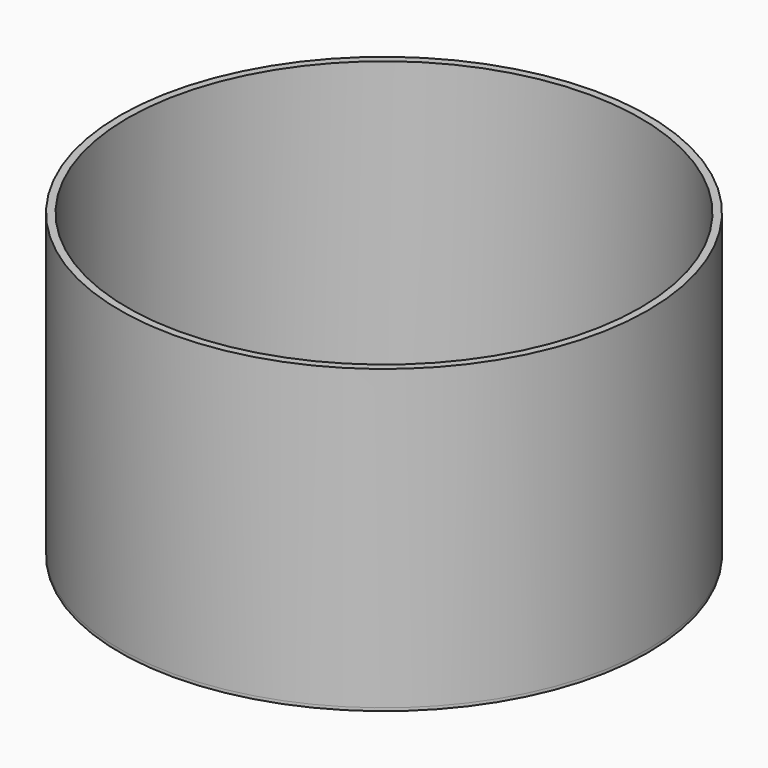
from build123d import *

# Parameters (mm, degrees)
F2_R     = 44.958
F3_DEPTH = 0.508
F4_R     = 44.958
F4_R_2   = 43.688
F5_DEPTH = 50.8


# Not quite as in the source:
# - the program builds the solid bodies; features that only make, move or delete a surface that nothing else refers to are left out


with BuildPart() as f3:
    # F2 (on Top) → F3 (new body)
    with BuildSketch(Plane.XY):
        Circle(F2_R)
    extrude(amount=-F3_DEPTH)

    # F4 (on Top) → F5 (join)
    with BuildSketch(Plane.XY):
        Circle(F4_R)
        Circle(F4_R_2, mode=Mode.SUBTRACT)
    extrude(amount=F5_DEPTH)


solid = f3.part
